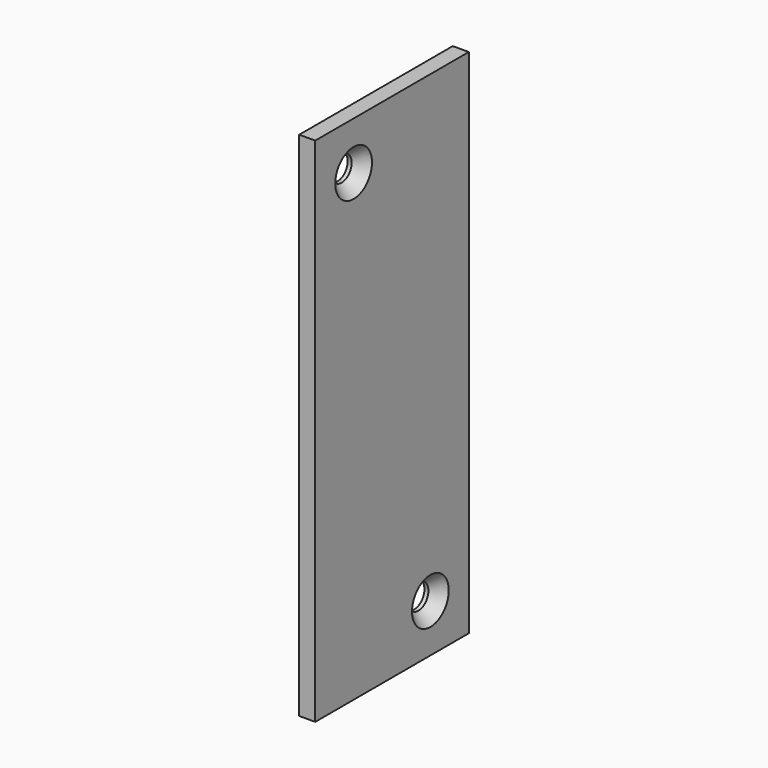
from build123d import *

# Parameters (mm, degrees)
F0_W           = 38.1
F0_H           = 101.6
F1_DEPTH       = 3.175
F3_D           = 4.9784
F3_CSINK_D     = 9.1186
F3_CSINK_ANGLE = 82


# Not quite as in the source:
# - a feature names something its author has since deleted; it is built from what else it names


with BuildPart() as f1:
    # F0 (on Right) → F1 (new body)
    with BuildSketch(Plane.YZ):
        Rectangle(F0_W, F0_H)
    extrude(amount=F1_DEPTH)

    # F3 (through all)
    with Locations(Plane.YZ.offset(3.175)):
        with Locations((-9.525, 41.275), (9.525, -41.275)):
            CounterSinkHole(F3_D / 2, F3_CSINK_D / 2, counter_sink_angle=F3_CSINK_ANGLE)


solid = f1.part
